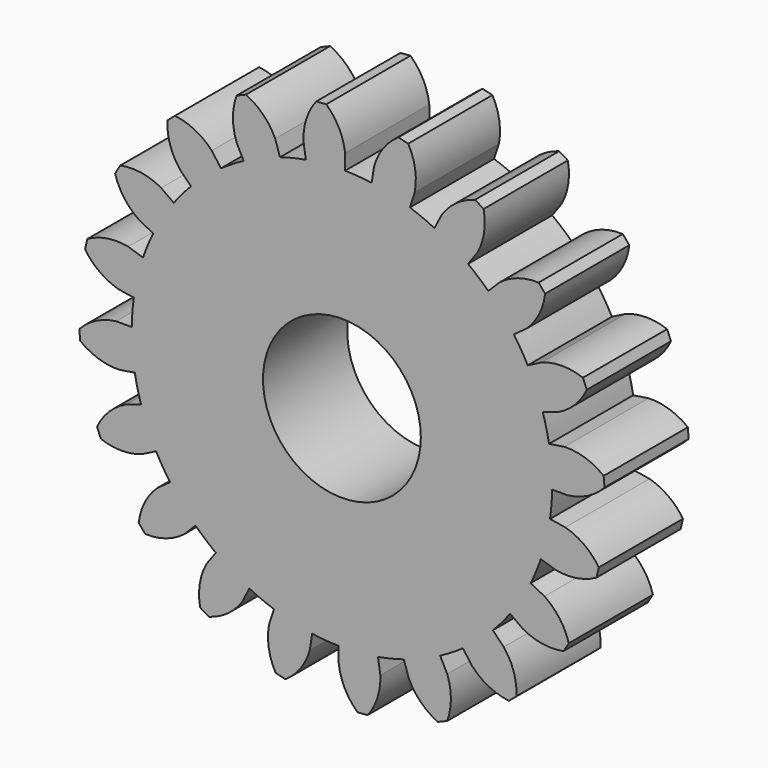
from build123d import *

# Parameters (mm, degrees)
F1_R     = 0.75
F2_DEPTH = 1
F3_COUNT = 20
F3_ANGLE = 342


# Not quite as in the source:
# - a feature names something its author has since deleted; it is built from what else it names


with BuildPart() as f2:
    # F1 (on Front) → F2 (new body)
    with BuildSketch(Plane.XZ):
        with BuildLine():
            ThreePointArc((-0.342416875, 1.9684396571), (-1.2860511428, -1.5290769955), (1.998, 0))
            ThreePointArc((1.998, 0), (1.4234609517, 1.4020566747), (0.0302693503, 1.9977706992))
            ThreePointArc((0.0302693503, 1.9977706992), (-0.1567612733, 1.9918408328), (-0.342416875, 1.9684396571))
        make_face()
        Circle(F1_R, mode=Mode.SUBTRACT)
        with BuildLine():
            ThreePointArc((-0.342416875, 1.9684396571), (-0.1567612733, 1.9918408328), (0.0302693503, 1.9977706992))
            Line((0.0302693503, 1.9977706992), (0.0302693503, 2.145667056))
            ThreePointArc((0.0302693503, 2.145667056), (-0.0277660563, 2.3365498257), (-0.1482087326, 2.4956029675))
            Line((-0.1482087326, 2.4956029675), (-0.244014278, 2.4880629076))
            ThreePointArc((-0.244014278, 2.4880629076), (-0.3380927119, 2.3121265883), (-0.3655529625, 2.1145151644))
            Line((-0.3655529625, 2.1145151644), (-0.342416875, 1.9684396571))
        make_face()
    extrude(amount=-F2_DEPTH)

    # F3: F2 ×20 about axis
    f3_axis = Axis((0, 0, 0), (0, -1, 0))


with BuildPart() as f2_1:
    add(f2.part)
    for i in range(1, F3_COUNT):
        add(f2.part.rotate(f3_axis, i * F3_ANGLE / (F3_COUNT - 1)))


solid = f2_1.part
